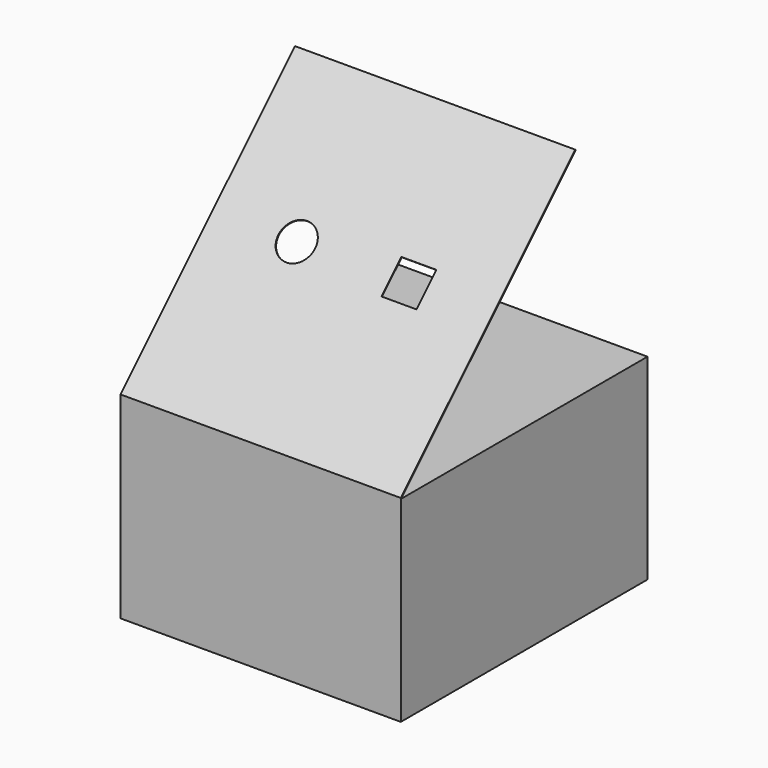
from build123d import *

# Parameters (mm, degrees)
F1_DEPTH = 63.5
F2_W     = 15.875
F2_H     = 15.875
F3_DEPTH = 0.4064


# Not quite as in the source:
# - the dataset's text gives a spline's control points without its knots; the knots are read off the source's solid


with BuildPart() as f1:
    # F0 (on Right) → F1 (new body, symmetric)
    with BuildSketch(Plane.YZ):
        Polygon((-139.7, 0), (0, 0), (0, 88.9), (-139.2936, 88.9), (-139.2936, 89.154), (-40.6298144724, 187.8177855276), (-40.9171826682, 188.1051537235), (-139.7, 89.3223363917), align=None)
    extrude(amount=F1_DEPTH, both=True)

    # F2 (on face) → F3 (cut, through all)
    with BuildSketch(Plane(origin=(0, -114.5111681959, 114.5111681959), x_dir=(1, 0, 0), z_dir=(0, -0.7071067812, 0.7071067812))):
        with Locations((25.435084784, 38.0925593219)):
            Rectangle(F2_W, F2_H)
        with BuildLine():
            add(Edge.make_bspline(
                [(-19.471708816, 43.9859181219), (-21.014403216, 45.5287903219), (-23.182750416, 46.4269343219), (-25.364915216, 46.4269343219)],
                knots=[7, 7, 7, 7, 8, 8, 8, 8], degree=3))
            add(Edge.make_bspline(
                [(-25.364915216, 46.4269343219), (-27.546648216, 46.4269343219), (-29.715351016, 45.5287903219), (-31.258045416, 43.9859181219)],
                knots=[0, 0, 0, 0, 1, 1, 1, 1], degree=3))
            add(Edge.make_bspline(
                [(-31.258045416, 43.9859181219), (-32.800790616, 42.4430205219), (-33.699290216, 40.2745209219), (-33.699290216, 38.0925593219), (-33.699290216, 35.9107755219), (-32.800790616, 33.7420981219), (-31.258045416, 32.1993529219)],
                knots=[1, 1, 1, 1, 2, 2, 2, 3, 3, 3, 3], degree=3))
            add(Edge.make_bspline(
                [(-31.258045416, 32.1993529219), (-29.715351016, 30.6563029219), (-27.546648216, 29.7581843219), (-25.364915216, 29.7581843219), (-23.182750416, 29.7581843219), (-21.014403216, 30.6563029219), (-19.471708816, 32.1993529219)],
                knots=[3, 3, 3, 3, 4, 4, 4, 5, 5, 5, 5], degree=3))
            add(Edge.make_bspline(
                [(-19.471708816, 32.1993529219), (-17.928658816, 33.7420981219), (-17.030540216, 35.9107755219), (-17.030540216, 38.0925593219), (-17.030540216, 40.2745209219), (-17.928658816, 42.4430205219), (-19.471708816, 43.9859181219)],
                knots=[5, 5, 5, 5, 6, 6, 6, 7, 7, 7, 7], degree=3))
        make_face()
    extrude(amount=-F3_DEPTH, mode=Mode.SUBTRACT)


solid = f1.part
